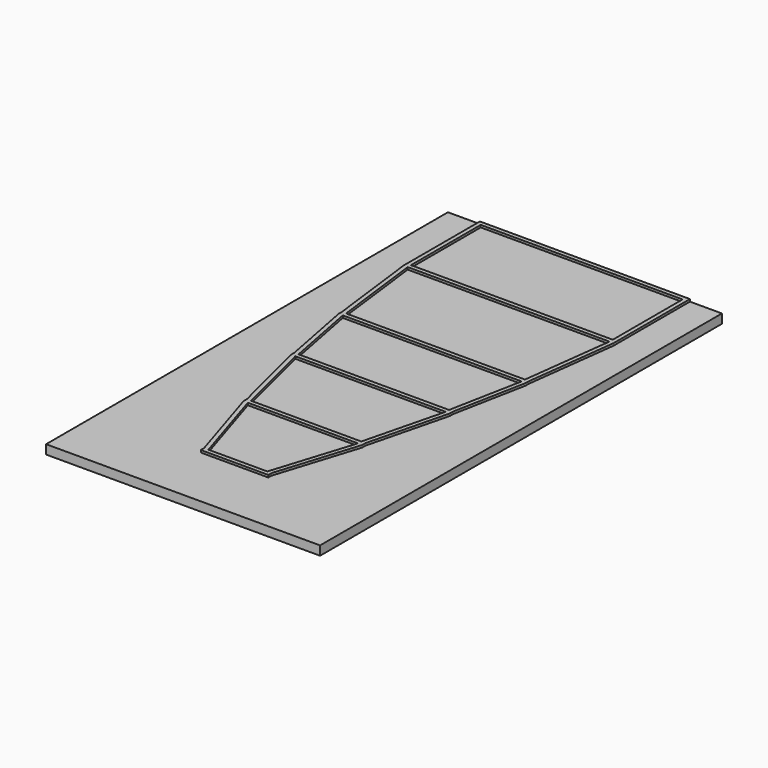
from build123d import *

# Parameters (mm, degrees)
F0_W     = 2210
F0_H     = 955
F0_W_2   = 45
F1_DEPTH = 100
F2_DEPTH = 125
F3_DEPTH = 125


# Not quite as in the source:
# - a feature names something its author has since deleted; it is built from what else it names


with BuildPart() as f1:
    # F0 (on Top) → F1 (new body)
    with BuildSketch(Plane.XY):
        Polygon((1500, -1587.5), (1500, 2912.5), (1150, 2912.5), (1150, 2867.5), (1150, 1912.5), (1150, 1867.5), (1025, 867.5), (1025, 822.5), (870, 22.5), (870, -22.5), (650, -902.5), (650, -947.5), (370, -1837.5), (370, -1882.5), (-370, -1882.5), (-370, -1837.5), (-650, -947.5), (-650, -902.5), (-870, -22.5), (-870, 22.5), (-1025, 822.5), (-1025, 867.5), (-1150, 1867.5), (-1150, 1912.5), (-1150, 2867.5), (-1150, 2912.5), (-1500, 2912.5), (-1500, -1587.5), (-1500, -2587.5), (1500, -2587.5), align=None)
        Polygon((322.8255446377, -1837.5), (602.8255446377, -947.5), (-602.8255446377, -947.5), (-322.8255446377, -1837.5), align=None)
        Polygon((-602.8255446377, -947.5), (-650, -947.5), (-370, -1837.5), (-322.8255446377, -1837.5), align=None)
        Polygon((370, -1837.5), (650, -947.5), (602.8255446377, -947.5), (322.8255446377, -1837.5), align=None)
        Polygon((603.6150617118, -902.5), (823.6150617118, -22.5), (-823.6150617118, -22.5), (-603.6150617118, -902.5), align=None)
        Polygon((-823.6150617118, -22.5), (-870, -22.5), (-650, -902.5), (-603.6150617118, -902.5), align=None)
        Polygon((870, -22.5), (870, 22.5), (824.1631523601, 22.5), (-824.1631523601, 22.5), (-870, 22.5), (-870, -22.5), (-823.6150617118, -22.5), (823.6150617118, -22.5), align=None)
        Polygon((650, -902.5), (870, -22.5), (823.6150617118, -22.5), (603.6150617118, -902.5), align=None)
        Polygon((870, 22.5), (1025, 822.5), (979.1631523601, 822.5), (824.1631523601, 22.5), align=None)
        Polygon((824.1631523601, 22.5), (979.1631523601, 822.5), (-979.1631523601, 822.5), (-824.1631523601, 22.5), align=None)
        Polygon((-979.1631523601, 822.5), (-1025, 822.5), (-870, 22.5), (-824.1631523601, 22.5), align=None)
        Polygon((1025, 822.5), (1025, 867.5), (979.6498001658, 867.5), (-979.6498001658, 867.5), (-1025, 867.5), (-1025, 822.5), (-979.1631523601, 822.5), (979.1631523601, 822.5), align=None)
        Polygon((979.6498001658, 867.5), (1104.6498001658, 1867.5), (-1104.6498001658, 1867.5), (-979.6498001658, 867.5), align=None)
        Polygon((1025, 867.5), (1150, 1867.5), (1104.6498001658, 1867.5), (979.6498001658, 867.5), align=None)
        Polygon((1150, 1867.5), (1150, 1912.5), (1105, 1912.5), (-1105, 1912.5), (-1150, 1912.5), (-1150, 1867.5), (-1104.6498001658, 1867.5), (1104.6498001658, 1867.5), align=None)
        Polygon((-1104.6498001658, 1867.5), (-1150, 1867.5), (-1025, 867.5), (-979.6498001658, 867.5), align=None)
        with Locations((0, 2390)):
            Rectangle(F0_W, F0_H)
        with Locations((1127.5, 2390)):
            Rectangle(F0_W_2, F0_H)
        Polygon((1150, 2867.5), (1150, 2912.5), (-1150, 2912.5), (-1150, 2867.5), (-1105, 2867.5), (1105, 2867.5), align=None)
        with Locations((-1127.5, 2390)):
            Rectangle(F0_W_2, F0_H)
        Polygon((650, -947.5), (650, -902.5), (603.6150617118, -902.5), (-603.6150617118, -902.5), (-650, -902.5), (-650, -947.5), (-602.8255446377, -947.5), (602.8255446377, -947.5), align=None)
        Polygon((370, -1882.5), (370, -1837.5), (322.8255446377, -1837.5), (-322.8255446377, -1837.5), (-370, -1837.5), (-370, -1882.5), align=None)
    extrude(amount=F1_DEPTH)

    # F0 (on Top) → F2 (join)
    with BuildSketch(Plane.XY):
        Polygon((1150, 1867.5), (1150, 1912.5), (1105, 1912.5), (-1105, 1912.5), (-1150, 1912.5), (-1150, 1867.5), (-1104.6498001658, 1867.5), (1104.6498001658, 1867.5), align=None)
        Polygon((1025, 822.5), (1025, 867.5), (979.6498001658, 867.5), (-979.6498001658, 867.5), (-1025, 867.5), (-1025, 822.5), (-979.1631523601, 822.5), (979.1631523601, 822.5), align=None)
        Polygon((870, -22.5), (870, 22.5), (824.1631523601, 22.5), (-824.1631523601, 22.5), (-870, 22.5), (-870, -22.5), (-823.6150617118, -22.5), (823.6150617118, -22.5), align=None)
        Polygon((650, -947.5), (650, -902.5), (603.6150617118, -902.5), (-603.6150617118, -902.5), (-650, -902.5), (-650, -947.5), (-602.8255446377, -947.5), (602.8255446377, -947.5), align=None)
        Polygon((370, -1882.5), (370, -1837.5), (322.8255446377, -1837.5), (-322.8255446377, -1837.5), (-370, -1837.5), (-370, -1882.5), align=None)
        Polygon((1150, 2867.5), (1150, 2912.5), (-1150, 2912.5), (-1150, 2867.5), (-1105, 2867.5), (1105, 2867.5), align=None)
    extrude(amount=F2_DEPTH)

    # F0 (on Top) → F3 (join)
    with BuildSketch(Plane.XY):
        Polygon((-602.8255446377, -947.5), (-650, -947.5), (-370, -1837.5), (-322.8255446377, -1837.5), align=None)
        Polygon((370, -1837.5), (650, -947.5), (602.8255446377, -947.5), (322.8255446377, -1837.5), align=None)
        Polygon((-823.6150617118, -22.5), (-870, -22.5), (-650, -902.5), (-603.6150617118, -902.5), align=None)
        Polygon((650, -902.5), (870, -22.5), (823.6150617118, -22.5), (603.6150617118, -902.5), align=None)
        Polygon((870, 22.5), (1025, 822.5), (979.1631523601, 822.5), (824.1631523601, 22.5), align=None)
        Polygon((-979.1631523601, 822.5), (-1025, 822.5), (-870, 22.5), (-824.1631523601, 22.5), align=None)
        Polygon((1025, 867.5), (1150, 1867.5), (1104.6498001658, 1867.5), (979.6498001658, 867.5), align=None)
        with Locations((1127.5, 2390)):
            Rectangle(F0_W_2, F0_H)
        with Locations((-1127.5, 2390)):
            Rectangle(F0_W_2, F0_H)
        Polygon((-1104.6498001658, 1867.5), (-1150, 1867.5), (-1025, 867.5), (-979.6498001658, 867.5), align=None)
    extrude(amount=F3_DEPTH)


solid = f1.part
